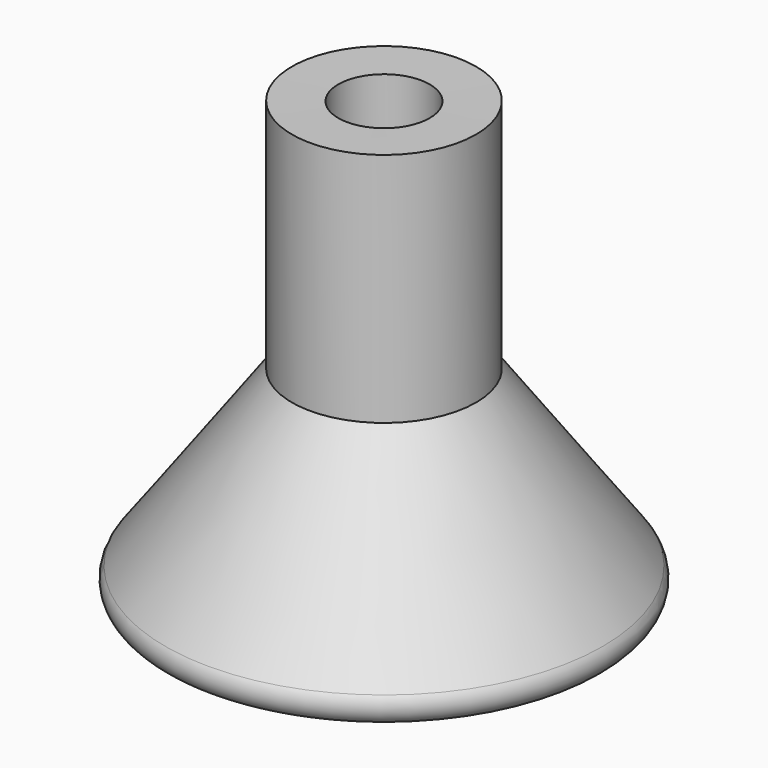
from build123d import *

# Parameters (mm, degrees)
F2_R     = 12.7
F3_DEPTH = 76.2
F4_R     = 5.08


# Not quite as in the source:
# - a feature names something its author has since deleted; it is built from what else it names


with BuildPart() as f1:
    # F0 (on Front) → F1 (revolve)
    with BuildSketch(Plane.XZ):
        Polygon((0, -45.9611259629), (66.641533635, -45.9611259629), (25.5837057043, 10.3556019993), (25.5837057043, 75.9213268757), (0, 75.5790621042), align=None)
    revolve(axis=Axis((0, 0, 14.8089680707), (0, 0, -1)))

    # F2 (on Top) → F3 (cut, symmetric)
    with BuildSketch(Plane.XY):
        Circle(F2_R)
    extrude(amount=F3_DEPTH, both=True, mode=Mode.SUBTRACT)

    # F4
    f4_edges = [f1.edges().sort_by_distance(p)[0] for p in [
        (-66.641534, 0, -45.961126),
    ]]
    fillet(f4_edges, radius=F4_R)


solid = f1.part
